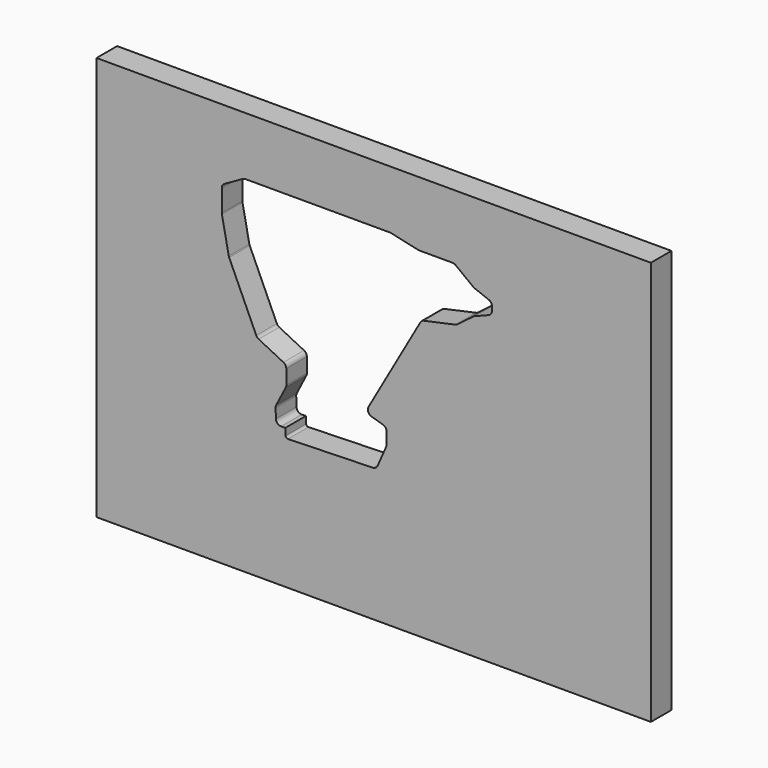
from build123d import *

# Parameters (mm, degrees)
F0_W     = 546.8174844539
F0_H     = 398.7210936817
F1_DEPTH = 25.4
F3_DEPTH = 25.401
F4_R     = 5.08
F5_R     = 2.159


# Not quite as in the source:
# - a feature names something its author has since deleted; it is built from what else it names


with BuildPart() as f1:
    # F0 (on Front) → F1 (new body)
    with BuildSketch(Plane.XZ):
        with Locations((480.6314062452, -83.1606246494)):
            Rectangle(F0_W, F0_H)
        Polygon((330.755193297, 46.4165987058), (352.6924322393, 58.7807495217), (497.1109463772, 58.7807495217), (525.0629135844, 52.5692068872), (560.0028810439, 52.5692068872), (579.4140003676, 37.8167783416), (597.2722044557, 30.8287886525), (597.2722044557, 19.9585742536), (579.4140003676, 12.9705761138), (562.3322031939, 0), (493.2287427939, -14.9813921496), (476.9234201392, -48.3684665562), (464.5003348701, -54.5800176413), (451.3007750821, -98.8373032779), (493.3564558907, -111.380243164), (493.3564558907, -127.5657196522), (483.1349796749, -150.8590341088), (393.7753742012, -153.3092504783), (393.5303500451, -144.3731980569), (384.284519278, -144.626716252), (383.8496065952, -128.7654126401), (394.4104195536, -108.2215374956), (394.4104195536, -64.4587469067), (400.6219790893, -38.8361145254), (368.0113337798, -22.5307876454), (337.8036322085, -13.9719399936), (330.755193297, 21.270351746), align=None, mode=Mode.SUBTRACT)
    extrude(amount=F1_DEPTH)

    # F2 (on face) → F3 (cut, through all)
    with BuildSketch(Plane.XZ.offset(25.4)):
        Polygon((527.7804729939, -7.4906960748), (337.8036322085, -13.9719399936), (365.5445277691, -75.1346200705), (401.7401635647, -93.1630060077), (472.3286154864, -105.1087732209), align=None)
    extrude(amount=-F3_DEPTH, mode=Mode.SUBTRACT)

    # F4
    f4_edges = [f1.edges().sort_by_distance(p)[0] for p in [
        (330.755193, -12.7, 21.270352),
        (330.755193, -12.7, 46.416599),
        (352.692432, -12.7, 58.78075),
        (337.803632, -12.7, -13.97194),
        (394.41042, -12.7, -108.221537),
        (383.849607, -12.7, -128.765413),
        (384.284519, -12.7, -144.626716),
        (483.13498, -12.7, -150.859034),
        (493.356456, -12.7, -127.56572),
        (562.332203, -12.7, 0),
        (579.414, -12.7, 12.970576),
        (597.272204, -12.7, 19.958574),
        (493.356456, -12.7, -111.380243),
        (525.062914, -12.7, 52.569207),
        (560.002881, -12.7, 52.569207),
        (579.414, -12.7, 37.816778),
        (597.272204, -12.7, 30.828789),
        (497.110946, -12.7, 58.78075),
        (365.544528, -12.7, -75.13462),
        (472.328615, -12.7, -105.108773),
        (394.41042, -12.7, -89.512194),
        (527.780473, -12.7, -7.490696),
    ]]
    fillet(f4_edges, radius=F4_R)

    # F5
    f5_edges = [f1.edges().sort_by_distance(p)[0] for p in [
        (393.775374, -12.7, -153.30925),
    ]]
    fillet(f5_edges, radius=F5_R)


solid = f1.part
